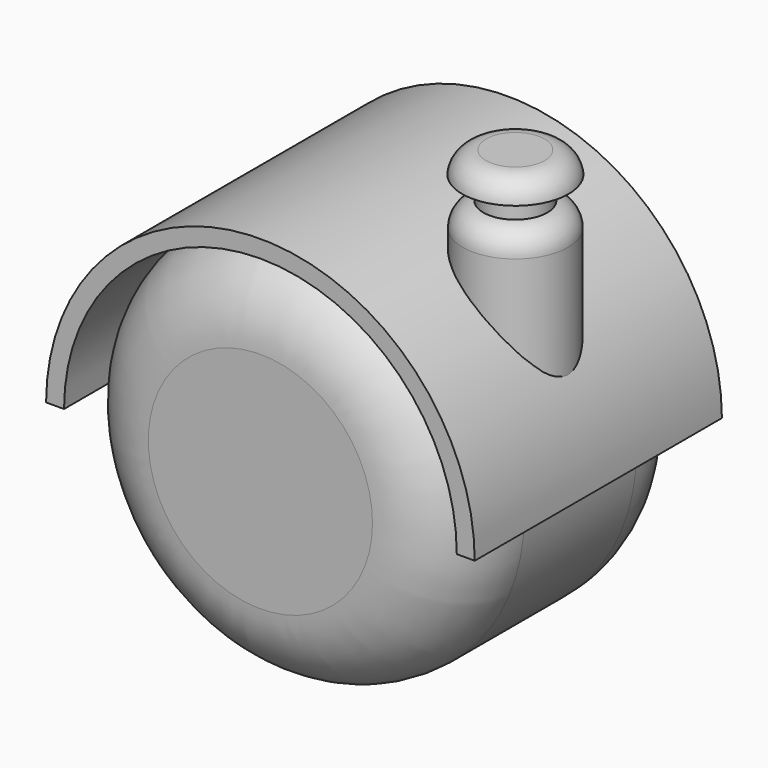
from build123d import *

# Parameters (mm, degrees)
F0_R      = 29.99994
F1_DEPTH  = 47.2000072
F4_R      = 8.0459114743
F5_DEPTH  = 35.56
F6_R      = 4.8880627921
F7_DEPTH  = 3.556
F8_R      = 8.1274992905
F9_DEPTH  = 3.302
F11_DEPTH = 47.2004644
F12_R     = 12.8774151417


# Not quite as in the source:
# - a fillet or chamfer that OpenCascade refuses, or shapes differently, is made with other operations: its cross-section is extruded or revolved along the edge and cut away or added
# - the program builds the solid bodies; features that only make, move or delete a surface that nothing else refers to are left out


with BuildPart() as f1:
    # F0 (on Front) → F1 (new body)
    with BuildSketch(Plane.XZ):
        Circle(F0_R)
    extrude(amount=F1_DEPTH)

    # F4 (on Top) → F5 (join)
    with BuildSketch(Plane.XY):
        with Locations((21.1084838957, -24.9004270881)):
            Circle(F4_R)
    extrude(amount=F5_DEPTH)

    # F6 (on face) → F7 (join)
    with BuildSketch(Plane.XY.offset(35.56)):
        with Locations((21.1084838957, -24.9004270881)):
            Circle(F6_R)
    extrude(amount=F7_DEPTH)

    # F8 (on face) → F9 (join)
    with BuildSketch(Plane.XY.offset(39.116)):
        with Locations((21.1084838957, -24.9004270881)):
            Circle(F8_R)
    extrude(amount=F9_DEPTH)

    # F12
    f12_edges = [f1.edges().sort_by_distance(p)[0] for p in [
        (-29.99994, 0, 0),
        (-29.99994, -47.200007, 0),
    ]]
    fillet(f12_edges, radius=F12_R)

    # F13: fillet of radius 3.6792614691 on 1 edges, made by hand

    # F13_s1 → F13_t2 (revolve, cut)
    with BuildSketch(Plane.XZ.offset(24.9004270881)):
        with BuildLine():
            ThreePointArc((29.1543953699, 31.9178723714), (28.2550061042, 34.3281162367), (25.9965466878, 35.56))
            Line((25.9965466878, 35.56), (26.0069749435, 35.6328425526))
            ThreePointArc((26.0069749435, 35.6328425526), (27.5754710288, 35.6335852294), (29.1543953699, 35.6335852294))
            Line((29.1543953699, 35.6335852294), (29.2279805993, 35.56))
            Line((29.2279805993, 35.56), (29.2279805993, 31.9178723714))
            Line((29.2279805993, 31.9178723714), (29.1543953699, 31.9178723714))
        make_face()
    revolve(axis=Axis((21.1084838957, -24.9004270881, 35.56), (0, 0, 1)), mode=Mode.SUBTRACT)

    # F14: fillet of radius 3.6792614691 on 1 edges, made by hand

    # F14_s1 → F14_t2 (revolve, cut)
    with BuildSketch(Plane.XZ.offset(24.9004270881)):
        with BuildLine():
            ThreePointArc((29.2359831862, 39.116), (28.0407566088, 41.4704969888), (25.576114508, 42.418))
            Line((25.576114508, 42.418), (29.2359831862, 42.418))
            Line((29.2359831862, 42.418), (29.2359831862, 39.116))
        make_face()
    revolve(axis=Axis((21.1084838957, -24.9004270881, 42.418), (0, 0, 1)), mode=Mode.SUBTRACT)


with BuildPart() as f11:
    # F10 (on face) → F11 (new body)
    with BuildSketch(Plane.XZ.offset(47.2000072)):
        with BuildLine():
            ThreePointArc((-29.99994, 0), (0, 29.99994), (29.99994, 0))
            Line((29.99994, 0), (32.74314, 0))
            ThreePointArc((32.74314, 0), (0, 32.6558421266), (-32.74314, 0))
            Line((-32.74314, 0), (-29.99994, 0))
        make_face()
    extrude(amount=-F11_DEPTH)


solid = Compound([f1.part, f11.part])
